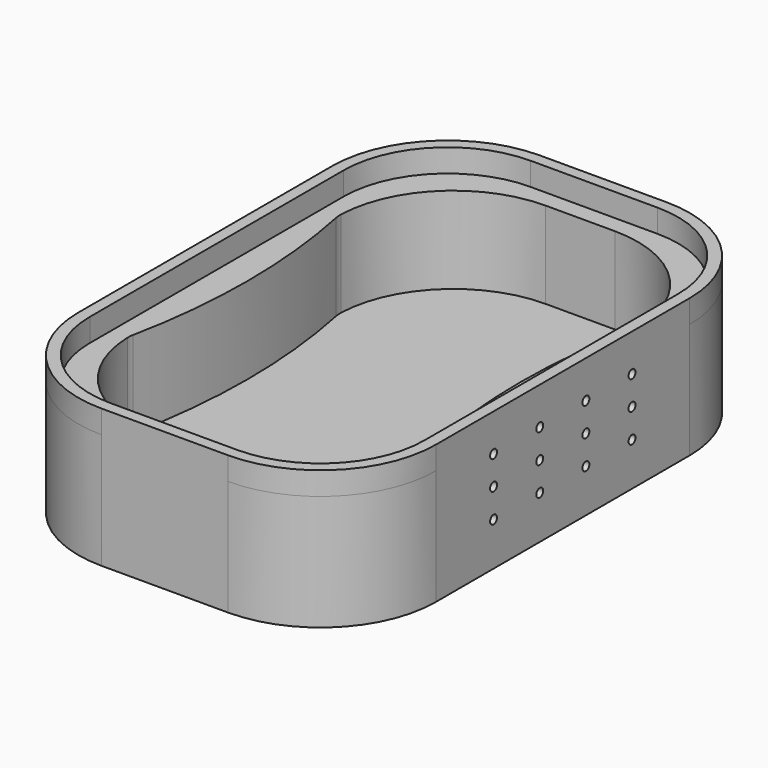
from build123d import *

# Parameters (mm, degrees)
F1_DEPTH       = 15
F3_W           = 61.9800009431
F3_H           = 95
F4_DEPTH       = 20
F6_R           = 20
F7_TEXT_SIZE   = 11.1111111111
F8_DEPTH       = 0.3
F9_TEXT_SIZE   = 2.7777777778
F9_TEXT_SIZE_2 = 4.5941832165
F10_DEPTH      = 0.2
F11_R          = 0.75
F12_DEPTH      = 25
F14_DEPTH      = 4


# Not quite as in the source:
# - Text() gives the source's letters only with a copy of the font that has no kerning and outlines rounded to 1/6400 em; it was checked with that copy


with BuildPart() as f1:
    # F0 (on Top) → F1 (new body)
    with BuildSketch(Plane.XY):
        with BuildLine():
            ThreePointArc((0.0099995284, 19.3676384362), (6.0832336959, 5.6360306448), (20, 0))
            Line((20, 0), (32, 0))
            ThreePointArc((32, 0), (45.9167663041, 5.6360306448), (51.9900004716, 19.3676384362))
            ThreePointArc((51.9900004716, 19.3676384362), (51.9745533731, 19.9489872725), (51.8917080486, 20.5246101825))
            ThreePointArc((51.8917080486, 20.5246101825), (49.6742773368, 42.5), (51.8917080486, 64.4753898175))
            ThreePointArc((51.8917080486, 64.4753898175), (51.9745533731, 65.0510127275), (51.9900004716, 65.6323615638))
            ThreePointArc((51.9900004716, 65.6323615638), (45.9167663041, 79.3639693552), (32, 85))
            Line((32, 85), (20, 85))
            ThreePointArc((20, 85), (6.0832336959, 79.3639693552), (0.0099995284, 65.6323615638))
            ThreePointArc((0.0099995284, 65.6323615638), (0.0254466269, 65.0510127275), (0.1082919514, 64.4753898175))
            ThreePointArc((0.1082919514, 64.4753898175), (2.3257226632, 42.5), (0.1082919514, 20.5246101825))
            ThreePointArc((0.1082919514, 20.5246101825), (0.0254466269, 19.9489872725), (0.0099995284, 19.3676384362))
        make_face()
    extrude(amount=-F1_DEPTH)


with BuildPart() as f4:
    # F3 (on offset) → F4 (new body)
    with BuildSketch(Plane.XY.offset(-20)):
        with Locations((26, 42.5)):
            Rectangle(F3_W, F3_H)
    extrude(amount=F4_DEPTH)

    # F5: cut F1
    add(f1.part, mode=Mode.SUBTRACT)

    # F6
    f6_edges = [f4.edges().sort_by_distance(p)[0] for p in [
        (-4.99, -5, -10),
        (-4.99, 90, -10),
        (56.99, 90, -10),
        (56.99, -5, -10),
    ]]
    fillet(f6_edges, radius=F6_R)

    # F7 (on face) → F8 (join)
    with BuildSketch(Plane(origin=(-4.9900004716, 0, 0), x_dir=(0, -1, 0), z_dir=(-1, 0, 0))):
        with Locations((-60.2417405907, -19.1019586176)):
            Text('Adrian', F7_TEXT_SIZE, font='Open Sans', text_align=(TextAlign.LEFT, TextAlign.BOTTOM))
    extrude(amount=F8_DEPTH)

    # F11 (on face) → F12 (cut)
    with BuildSketch(Plane.YZ.offset(56.9900004716)):
        with Locations((27.5, -12.5)):
            Circle(F11_R)
        with Locations((27.5, -7.5)):
            Circle(F11_R)
        with Locations((27.5, -2.5)):
            Circle(F11_R)
        with Locations((37.5, -12.5)):
            Circle(F11_R)
        with Locations((37.5, -7.5)):
            Circle(F11_R)
        with Locations((37.5, -2.5)):
            Circle(F11_R)
        with Locations((47.5, -12.5)):
            Circle(F11_R)
        with Locations((47.5, -7.5)):
            Circle(F11_R)
        with Locations((47.5, -2.5)):
            Circle(F11_R)
        with Locations((57.5, -12.5)):
            Circle(F11_R)
        with Locations((57.5, -7.5)):
            Circle(F11_R)
        with Locations((57.5, -2.5)):
            Circle(F11_R)
    extrude(amount=-F12_DEPTH, mode=Mode.SUBTRACT)

    # F13 (on face) → F14 (join)
    with BuildSketch(Plane.XY):
        with BuildLine():
            ThreePointArc((-4.9900004716, 15), (0.8678639047, 0.8578643763), (15.0099995284, -5))
            Line((15.0099995284, -5), (36.9900004716, -5))
            ThreePointArc((36.9900004716, -5), (51.1321360953, 0.8578643763), (56.9900004716, 15))
            Line((56.9900004716, 15), (56.9900004716, 70))
            ThreePointArc((56.9900004716, 70), (51.1321360953, 84.1421356237), (36.9900004716, 90))
            Line((36.9900004716, 90), (15.0099995284, 90))
            ThreePointArc((15.0099995284, 90), (0.8678639047, 84.1421356237), (-4.9900004716, 70))
            Line((-4.9900004716, 70), (-4.9900004716, 15))
        make_face()
        with BuildLine():
            ThreePointArc((-2.9900004716, 70), (2.2820774671, 82.7279220614), (15.0099995284, 88))
            Line((15.0099995284, 88), (36.9900004716, 88))
            ThreePointArc((36.9900004716, 88), (49.7179225329, 82.7279220614), (54.9900004716, 70))
            Line((54.9900004716, 70), (54.9900004716, 15))
            ThreePointArc((54.9900004716, 15), (49.7179225329, 2.2720779386), (36.9900004716, -3))
            Line((36.9900004716, -3), (15.0099995284, -3))
            ThreePointArc((15.0099995284, -3), (2.2820774671, 2.2720779386), (-2.9900004716, 15))
            Line((-2.9900004716, 15), (-2.9900004716, 70))
        make_face(mode=Mode.SUBTRACT)
    extrude(amount=F14_DEPTH)


with BuildPart() as f10:
    # F9 (on face) → F10 (new body)
    with BuildSketch(Plane(origin=(0, 0, -20), x_dir=(1, 0, 0), z_dir=(0, 0, -1))):
        with Locations((14.7478639047, -87.9978525095)):
            Text('MADE IN MEXICO', F9_TEXT_SIZE, font='Open Sans', text_align=(TextAlign.LEFT, TextAlign.BOTTOM))
        with Locations((24.1522421922, -84.9978525095)):
            Text('Ω', F9_TEXT_SIZE_2, font='Open Sans', text_align=(TextAlign.LEFT, TextAlign.BOTTOM))
    extrude(amount=-F10_DEPTH)


solid = Compound([f4.part, f10.part])
